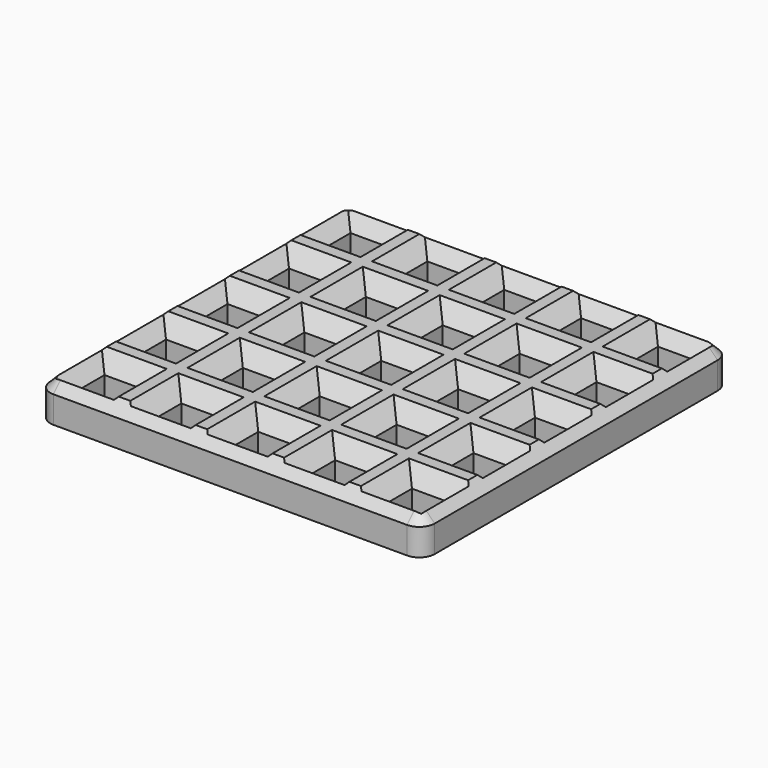
from build123d import *

# Parameters (mm, degrees)
F0_W         = 50
F0_H         = 50
F0_W_2       = 4.5
F0_H_2       = 4.5
F1_DEPTH     = 5
F2_SIZE      = 2
F3_R         = 2
F4_T1_DEPTH  = 46
F4_T3_DEPTH  = 46
F4_T6_ANGLE  = 90
F4_T8_ANGLE  = 90
F4_T10_ANGLE = 90
F4_T12_ANGLE = 90


# Not quite as in the source:
# - a fillet or chamfer that OpenCascade refuses, or shapes differently, is made with other operations: its cross-section is extruded or revolved along the edge and cut away or added


with BuildPart() as f1:
    # F0 (on Top) → F1 (new body)
    with BuildSketch(Plane.XY):
        Rectangle(F0_W, F0_H)
        with Locations((-19.95, -19.95)):
            Rectangle(F0_W_2, F0_H_2, mode=Mode.SUBTRACT)
        with Locations((-9.95, -19.95)):
            Rectangle(F0_W_2, F0_H_2, mode=Mode.SUBTRACT)
        with Locations((-19.95, -9.95)):
            Rectangle(F0_W_2, F0_H_2, mode=Mode.SUBTRACT)
        with Locations((-9.95, -9.95)):
            Rectangle(F0_W_2, F0_H_2, mode=Mode.SUBTRACT)
        with Locations((0.05, -19.95)):
            Rectangle(F0_W_2, F0_H_2, mode=Mode.SUBTRACT)
        with Locations((10.05, -19.95)):
            Rectangle(F0_W_2, F0_H_2, mode=Mode.SUBTRACT)
        with Locations((20.05, -19.95)):
            Rectangle(F0_W_2, F0_H_2, mode=Mode.SUBTRACT)
        with Locations((0.05, -9.95)):
            Rectangle(F0_W_2, F0_H_2, mode=Mode.SUBTRACT)
        with Locations((10.05, -9.95)):
            Rectangle(F0_W_2, F0_H_2, mode=Mode.SUBTRACT)
        with Locations((20.05, -9.95)):
            Rectangle(F0_W_2, F0_H_2, mode=Mode.SUBTRACT)
        with Locations((-19.95, 0.05)):
            Rectangle(F0_W_2, F0_H_2, mode=Mode.SUBTRACT)
        with Locations((-19.95, 10.05)):
            Rectangle(F0_W_2, F0_H_2, mode=Mode.SUBTRACT)
        with Locations((-9.95, 0.05)):
            Rectangle(F0_W_2, F0_H_2, mode=Mode.SUBTRACT)
        with Locations((-9.95, 10.05)):
            Rectangle(F0_W_2, F0_H_2, mode=Mode.SUBTRACT)
        with Locations((-19.95, 20.05)):
            Rectangle(F0_W_2, F0_H_2, mode=Mode.SUBTRACT)
        with Locations((-9.95, 20.05)):
            Rectangle(F0_W_2, F0_H_2, mode=Mode.SUBTRACT)
        with Locations((0.05, 0.05)):
            Rectangle(F0_W_2, F0_H_2, mode=Mode.SUBTRACT)
        with Locations((10.05, 0.05)):
            Rectangle(F0_W_2, F0_H_2, mode=Mode.SUBTRACT)
        with Locations((0.05, 10.05)):
            Rectangle(F0_W_2, F0_H_2, mode=Mode.SUBTRACT)
        with Locations((10.05, 10.05)):
            Rectangle(F0_W_2, F0_H_2, mode=Mode.SUBTRACT)
        with Locations((20.05, 0.05)):
            Rectangle(F0_W_2, F0_H_2, mode=Mode.SUBTRACT)
        with Locations((20.05, 10.05)):
            Rectangle(F0_W_2, F0_H_2, mode=Mode.SUBTRACT)
        with Locations((0.05, 20.05)):
            Rectangle(F0_W_2, F0_H_2, mode=Mode.SUBTRACT)
        with Locations((10.05, 20.05)):
            Rectangle(F0_W_2, F0_H_2, mode=Mode.SUBTRACT)
        with Locations((20.05, 20.05)):
            Rectangle(F0_W_2, F0_H_2, mode=Mode.SUBTRACT)
    extrude(amount=-F1_DEPTH)

    # F2
    f2_edges = [f1.edges().sort_by_distance(p)[0] for p in [
        (-22.2, -9.95, 0),
        (-22.2, -19.95, 0),
        (-19.95, -22.2, 0),
        (-17.7, -19.95, 0),
        (-19.95, -17.7, 0),
        (-17.7, -9.95, 0),
        (-19.95, -7.7, 0),
        (-19.95, 2.3, 0),
        (-22.2, 0.05, 0),
        (-9.95, -2.2, 0),
        (-9.95, 2.3, 0),
        (-12.2, 0.05, 0),
        (-7.7, 0.05, 0),
        (-9.95, -7.7, 0),
        (-9.95, -12.2, 0),
        (-12.2, -9.95, 0),
        (-7.7, -9.95, 0),
        (-9.95, -17.7, 0),
        (-12.2, -19.95, 0),
        (-9.95, -22.2, 0),
        (-7.7, -19.95, 0),
        (-2.2, -19.95, 0),
        (0.05, -17.7, 0),
        (0.05, -22.2, 0),
        (2.3, -9.95, 0),
        (0.05, -7.7, 0),
        (-2.2, -9.95, 0),
        (0.05, -12.2, 0),
        (0.05, 2.3, 0),
        (-2.2, 0.05, 0),
        (0.05, -2.2, 0),
        (2.3, 0.05, 0),
        (0.05, 7.8, 0),
        (0.05, 12.3, 0),
        (-2.2, 10.05, 0),
        (-7.7, 10.05, 0),
        (-9.95, 12.3, 0),
        (-12.2, 10.05, 0),
        (-9.95, 7.8, 0),
        (-17.7, 10.05, 0),
        (-19.95, 12.3, 0),
        (-22.2, 10.05, 0),
        (-19.95, 7.8, 0),
        (-22.2, 20.05, 0),
        (-19.95, 22.3, 0),
        (-19.95, 17.8, 0),
        (-17.7, 20.05, 0),
        (-9.95, 22.3, 0),
        (-12.2, 20.05, 0),
        (-9.95, 17.8, 0),
        (-7.7, 20.05, 0),
        (0.05, 22.3, 0),
        (0.05, 17.8, 0),
        (-2.2, 20.05, 0),
        (2.3, 20.05, 0),
        (10.05, 12.3, 0),
        (7.8, 10.05, 0),
        (10.05, 7.8, 0),
        (12.3, 10.05, 0),
        (10.05, 22.3, 0),
        (7.8, 20.05, 0),
        (10.05, 17.8, 0),
        (12.3, 20.05, 0),
        (17.8, 20.05, 0),
        (20.05, 22.3, 0),
        (22.3, 20.05, 0),
        (20.05, 17.8, 0),
        (20.05, 12.3, 0),
        (17.8, 10.05, 0),
        (22.3, 10.05, 0),
        (20.05, 7.8, 0),
        (20.05, 2.3, 0),
        (7.8, 0.05, 0),
        (10.05, -2.2, 0),
        (12.3, 0.05, 0),
        (10.05, 2.3, 0),
        (17.8, 0.05, 0),
        (20.05, -2.2, 0),
        (22.3, 0.05, 0),
        (20.05, -7.7, 0),
        (10.05, -7.7, 0),
        (7.8, -9.95, 0),
        (10.05, -17.7, 0),
        (7.8, -19.95, 0),
        (17.8, -9.95, 0),
        (10.05, -12.2, 0),
        (20.05, -17.7, 0),
        (17.8, -19.95, 0),
        (20.05, -22.2, 0),
        (22.3, -19.95, 0),
        (10.05, -22.2, 0),
        (22.3, -9.95, 0),
        (20.05, -12.2, 0),
        (-19.95, -12.2, 0),
        (-19.95, -2.2, 0),
        (-17.7, 0.05, 0),
        (2.3, -19.95, 0),
        (12.3, -9.95, 0),
        (12.3, -19.95, 0),
        (2.3, 10.05, 0),
    ]]
    chamfer(f2_edges, length=F2_SIZE)

    # F3
    f3_edges = [f1.edges().sort_by_distance(p)[0] for p in [
        (25, 25, -2.5),
        (25, -25, -2.5),
        (-25, -25, -2.5),
        (-25, 25, -2.5),
    ]]
    fillet(f3_edges, radius=F3_R)

    # F4: chamfer of 1.5 on 4 edges, made by hand

    # F4_s2 → F4_t1 (cut)
    with BuildSketch(Plane.YZ.offset(-23)):
        Polygon((25, -1.5), (23.5, 0), (25, 0), align=None)
        Polygon((-25, -1.5), (-23.5, 0), (-25, 0), align=None)
    extrude(amount=F4_T1_DEPTH, mode=Mode.SUBTRACT)

    # F4_s4 → F4_t3 (cut)
    with BuildSketch(Plane.XZ.offset(-23)):
        Polygon((25, -1.5), (23.5, 0), (25, 0), align=None)
        Polygon((-25, -1.5), (-23.5, 0), (-25, 0), align=None)
    extrude(amount=F4_T3_DEPTH, mode=Mode.SUBTRACT)

    # F4_s5 → F4_t6 (revolve, cut)
    with BuildSketch(Plane.YZ.offset(-23)):
        Polygon((25, -1.5), (23.5, 0), (25, 0), align=None)
    revolve(axis=Axis((-23, 23, 0), (0, 0, 1)), revolution_arc=F4_T6_ANGLE, mode=Mode.SUBTRACT)

    # F4_s7 → F4_t8 (revolve, cut)
    with BuildSketch(Plane.XZ.offset(23)):
        Polygon((-25, -1.5), (-23.5, 0), (-25, 0), align=None)
    revolve(axis=Axis((-23, -23, 0), (0, 0, 1)), revolution_arc=F4_T8_ANGLE, mode=Mode.SUBTRACT)

    # F4_s9 → F4_t10 (revolve, cut)
    with BuildSketch(Plane.XZ.offset(23)):
        Polygon((25, -1.5), (23.5, 0), (25, 0), align=None)
    revolve(axis=Axis((23, -23, 0), (0, 0, -1)), revolution_arc=F4_T10_ANGLE, mode=Mode.SUBTRACT)

    # F4_s11 → F4_t12 (revolve, cut)
    with BuildSketch(Plane.XZ.offset(-23)):
        Polygon((25, -1.5), (23.5, 0), (25, 0), align=None)
    revolve(axis=Axis((23, 23, 0), (0, 0, 1)), revolution_arc=F4_T12_ANGLE, mode=Mode.SUBTRACT)


solid = f1.part
